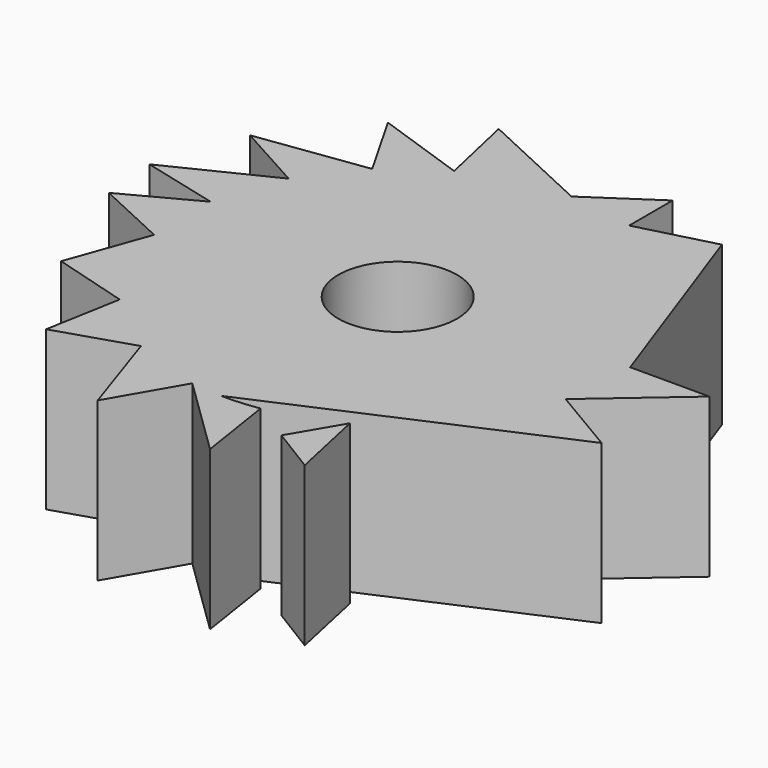
from build123d import *

# Parameters (mm, degrees)
F0_R     = 9.5147098481
F1_DEPTH = 25.4


with BuildPart() as f1:
    # F0 (on Top) → F1 (new body)
    with BuildSketch(Plane.XY):
        with BuildLine():
            ThreePointArc((33.7113661444, -8.521701965), (34.5056466306, -4.2937119493), (34.7717645756, 0))
            ThreePointArc((34.7717645756, 0), (34.7335993542, 1.6287073412), (34.6191874697, 3.253839369))
            Line((34.6191874697, 3.253839369), (28.8855670333, 19.357159628))
            ThreePointArc((28.8855670333, 19.357159628), (20.8860262727, 27.8001711908), (10.5496581318, 33.1327681458))
            ThreePointArc((10.5496581318, 33.1327681458), (5.3381081878, 34.3595723588), (4.9e-09, 34.7717645756))
            ThreePointArc((4.9e-09, 34.7717645756), (-8.1039598603, 33.8142195871), (-15.7615859684, 30.9943223746))
            ThreePointArc((-15.7615859684, 30.9943223746), (-20.1633398845, 28.3287016364), (-24.123479709, 25.0426304216))
            ThreePointArc((-24.123479709, 25.0426304216), (-27.7114808583, 21.003557802), (-30.630509106, 16.457445841))
            ThreePointArc((-30.630509106, 16.457445841), (-32.9437975869, 11.1257274932), (-34.3367194248, 5.4831843706))
            ThreePointArc((-34.3367194248, 5.4831843706), (-34.7710267297, -0.2265212223), (-34.2623659277, -5.930083704))
            ThreePointArc((-34.2623659277, -5.930083704), (-31.5524748858, -14.6122188692), (-26.6838149969, -22.2946098623))
            ThreePointArc((-26.6838149969, -22.2946098623), (-22.0925138505, -26.851376938), (-16.7366261479, -30.47886082))
            ThreePointArc((-16.7366261479, -30.47886082), (-11.2410746557, -32.9046174919), (-5.4100284558, -34.348321703))
            ThreePointArc((-5.4100284558, -34.348321703), (-2.9714241062, -34.6445702886), (-0.5179892362, -34.7679061615))
            Line((-0.5179892362, -34.7679061615), (25.9024363536, -23.1978318524))
            ThreePointArc((25.9024363536, -23.1978318524), (30.6968819131, -16.3333111315), (33.7113661444, -8.521701965))
        make_face()
        Circle(F0_R, mode=Mode.SUBTRACT)
        with BuildLine():
            Line((-45.7841467777, -0.5879337581), (-34.2623659277, -5.930083704))
            ThreePointArc((-34.2623659277, -5.930083704), (-34.7710267297, -0.2265212223), (-34.3367194248, 5.4831843706))
            Line((-34.3367194248, 5.4831843706), (-45.7841467777, -0.5879337581))
        make_face()
        with BuildLine():
            Line((-38.8848297568, -18.7696646387), (-26.6838149969, -22.2946098623))
            ThreePointArc((-26.6838149969, -22.2946098623), (-31.5524748858, -14.6122188692), (-34.2623659277, -5.930083704))
            Line((-34.2623659277, -5.930083704), (-38.8848297568, -18.7696646387))
        make_face()
        with BuildLine():
            Line((-28.8354200673, -34.3401022908), (-16.7366261479, -30.47886082))
            ThreePointArc((-16.7366261479, -30.47886082), (-22.0925138505, -26.851376938), (-26.6838149969, -22.2946098623))
            Line((-26.6838149969, -22.2946098623), (-28.8354200673, -34.3401022908))
        make_face()
        with BuildLine():
            Line((-11.7643075513, -45.344372684), (-5.4100284558, -34.348321703))
            ThreePointArc((-5.4100284558, -34.348321703), (-11.2410746557, -32.9046174919), (-16.7366261479, -30.47886082))
            Line((-16.7366261479, -30.47886082), (-11.7643075513, -45.344372684))
        make_face()
        with BuildLine():
            ThreePointArc((5.5066084769, -34.3329706665), (2.5037716955, -34.6815042782), (-0.5179892362, -34.7679061615))
            Line((-0.5179892362, -34.7679061615), (6.1559116798, -38.5238970706))
            Line((6.1559116798, -38.5238970706), (5.5066084769, -34.3329706665))
        make_face()
        with BuildLine():
            Line((6.1559116798, -38.5238970706), (-0.5179892362, -34.7679061615))
            ThreePointArc((-0.5179892362, -34.7679061615), (-2.9714241062, -34.6445702886), (-5.4100284558, -34.348321703))
            Line((-5.4100284558, -34.348321703), (7.4510303863, -46.8832385297))
            Line((7.4510303863, -46.8832385297), (6.1559116798, -38.5238970706))
        make_face()
        with BuildLine():
            Line((44.63919633, -14.992600468), (33.7113661444, -8.521701965))
            ThreePointArc((33.7113661444, -8.521701965), (30.6968819131, -16.3333111315), (25.9024363536, -23.1978318524))
            Line((25.9024363536, -23.1978318524), (44.63919633, -14.992600468))
        make_face()
        with BuildLine():
            ThreePointArc((34.6191874697, 3.253839369), (34.7335993542, 1.6287073412), (34.7717645756, 0))
            ThreePointArc((34.7717645756, 0), (34.5056466306, -4.2937119493), (33.7113661444, -8.521701965))
            Line((33.7113661444, -8.521701965), (47.3191874697, 3.253839369))
            Line((47.3191874697, 3.253839369), (34.6191874697, 3.253839369))
        make_face()
        with BuildLine():
            ThreePointArc((10.5496581318, 33.1327681458), (20.8860262727, 27.8001711908), (28.8855670333, 19.357159628))
            Line((28.8855670333, 19.357159628), (22.8358637772, 36.3482231429))
            Line((22.8358637772, 36.3482231429), (10.5496581318, 33.1327681458))
        make_face()
        with BuildLine():
            ThreePointArc((4.9e-09, 34.7717645756), (5.3381081878, 34.3595723588), (10.5496581318, 33.1327681458))
            Line((10.5496581318, 33.1327681458), (10.5496581218, 41.8424585666))
            Line((10.5496581218, 41.8424585666), (0, 34.7717645756))
        make_face()
        with BuildLine():
            ThreePointArc((-15.7615859684, 30.9943223746), (-8.1039598603, 33.8142195871), (4.9e-09, 34.7717645756))
            Line((0, 34.7717645756), (-18.5446361736, 43.3856351201))
            Line((-18.5446361736, 43.3856351201), (-15.7615859684, 30.9943223746))
        make_face()
        with BuildLine():
            ThreePointArc((-24.123479709, 25.0426304216), (-20.1633398845, 28.3287016364), (-15.7615859684, 30.9943223746))
            Line((-15.7615859684, 30.9943223746), (-30.4257869342, 36.0685509564))
            Line((-30.4257869342, 36.0685509564), (-24.123479709, 25.0426304216))
        make_face()
        with BuildLine():
            ThreePointArc((-30.630509106, 16.457445841), (-27.7114808583, 21.003557802), (-24.123479709, 25.0426304216))
            Line((-24.123479709, 25.0426304216), (-41.7405566495, 22.6102373684))
            Line((-41.7405566495, 22.6102373684), (-30.630509106, 16.457445841))
        make_face()
        with BuildLine():
            ThreePointArc((-34.3367194248, 5.4831843706), (-32.9437975869, 11.1257274932), (-30.630509106, 16.457445841))
            Line((-30.630509106, 16.457445841), (-46.6459102761, 8.6094953897))
            Line((-46.6459102761, 8.6094953897), (-34.3367194248, 5.4831843706))
        make_face()
    extrude(amount=F1_DEPTH)


with BuildPart() as f1b:
    # F0 (on Top) → F1, piece 2 (new body)
    with BuildSketch(Plane.XY):
        Polygon((19.4229201156, -42.8915085923), (16.7366261479, -30.47886082), (12.0884100824, -38.3807816184), align=None)
    extrude(amount=F1_DEPTH)


solid = Compound([f1.part, f1b.part])
